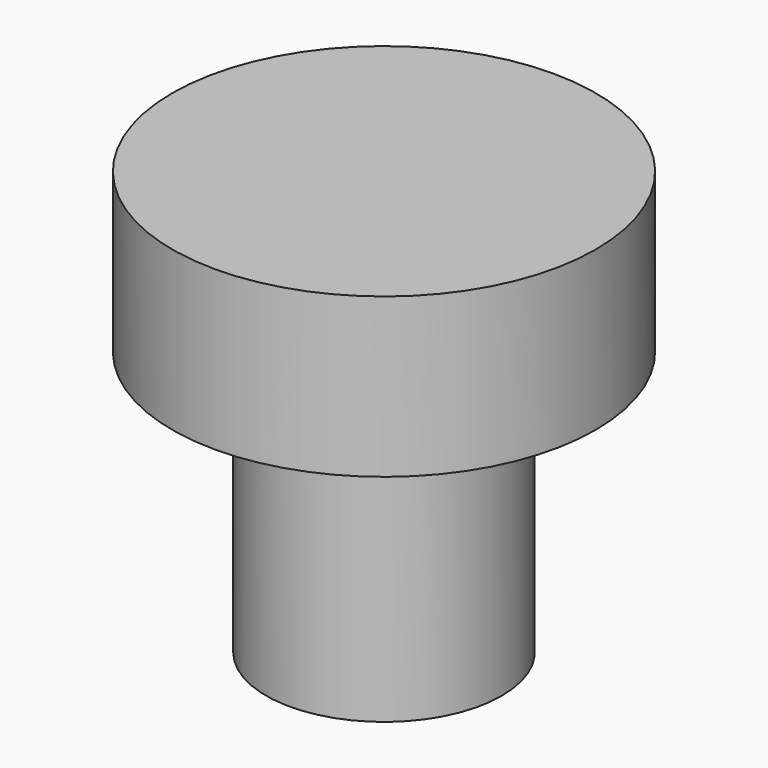
from build123d import *

# Parameters (mm, degrees)
F0_R     = 4.45
F0_R_2   = 3.95
F1_DEPTH = 8
F2_R     = 4.45
F3_DEPTH = 2
F4_R     = 8
F5_DEPTH = 6


# Not quite as in the source:
# - a feature names something its author has since deleted; it is built from what else it names


with BuildPart() as f1:
    # F0 (on Top) → F1 (new body)
    with BuildSketch(Plane.XY):
        Circle(F0_R)
        Circle(F0_R_2, mode=Mode.SUBTRACT)
    extrude(amount=F1_DEPTH)

    # F2 (on face) → F3 (join)
    with BuildSketch(Plane.XY.offset(8)):
        Circle(F2_R)
    extrude(amount=F3_DEPTH)

    # F4 (on face) → F5 (join)
    with BuildSketch(Plane.XY.offset(10)):
        Circle(F4_R)
    extrude(amount=F5_DEPTH)


solid = f1.part
